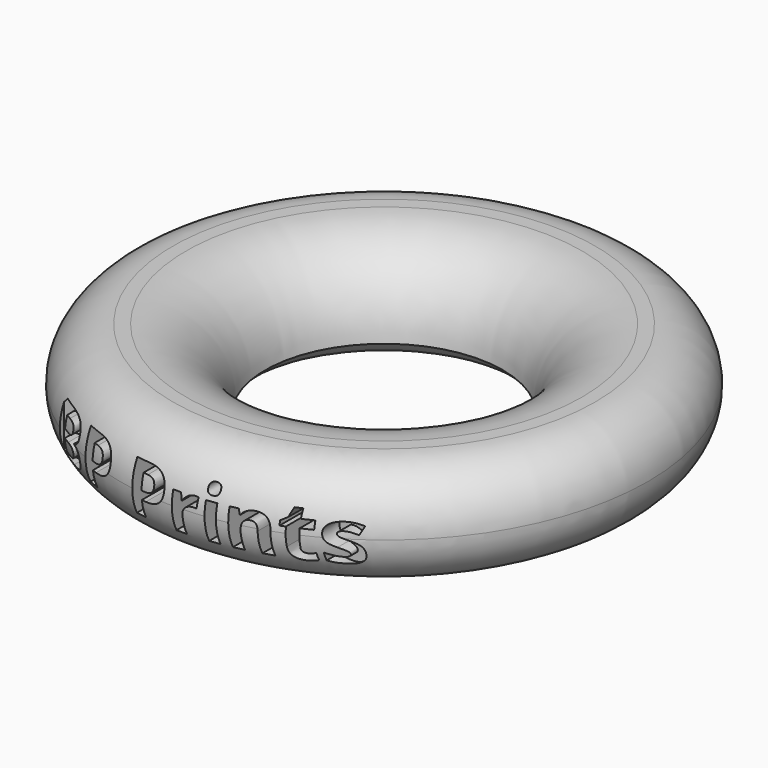
from build123d import *

# Parameters (mm, degrees)
F0_R         = 20
F0_R_2       = 9
F1_DEPTH     = 8
F2_R         = 6
F4_R         = 3.99999
F6_TEXT_SIZE = 5.223251944
F7_DEPTH     = 4


# Not quite as in the source:
# - a fillet or chamfer that OpenCascade refuses, or shapes differently, is made with other operations: its cross-section is extruded or revolved along the edge and cut away or added
# - a fillet or chamfer is up to 0.001 mm smaller than in the source, because OpenCascade refuses the exact size
# - Text() gives the source's letters only with a copy of the font that has no kerning and outlines rounded to 1/6400 em; it was checked with that copy


with BuildPart() as f1:
    # F0 (on Top) → F1 (new body)
    with BuildSketch(Plane.XY):
        Circle(F0_R)
        Circle(F0_R_2, mode=Mode.SUBTRACT)
    extrude(amount=F1_DEPTH)

    # F2
    f2_edges = [f1.edges().sort_by_distance(p)[0] for p in [
        (-9, 0, 8),
    ]]
    fillet(f2_edges, radius=F2_R)

    # F3: fillet of radius 6 on 1 edges, made by hand

    # F3_s1 → F3_t2 (revolve, cut)
    with BuildSketch(Plane.XZ):
        with BuildLine():
            ThreePointArc((9, 2), (11.0226462122, 0.5227744249), (13.472135955, 0))
            Line((13.472135955, 0), (9, 0))
            Line((9, 0), (9, 2))
        make_face()
    revolve(axis=Axis((0, 0, 0), (0, 0, 1)), mode=Mode.SUBTRACT)

    # F4 (radius 4 in the source; OpenCascade refuses exactly that, so slightly less here)
    f4_edges = [f1.edges().sort_by_distance(p)[0] for p in [
        (-20, 0, 8),
        (-20, 0, 0),
    ]]
    fillet(f4_edges, radius=F4_R)

    # F6 (on offset) → F7 (cut)
    with BuildSketch(Plane.XZ.offset(20)):
        with Locations((-11.9143192977, 2.1758442745)):
            Text('BP Prints', F6_TEXT_SIZE, font='Open Sans', font_style=FontStyle.BOLD, text_align=(TextAlign.LEFT, TextAlign.BOTTOM))
    extrude(amount=-F7_DEPTH, mode=Mode.SUBTRACT)


solid = f1.part
